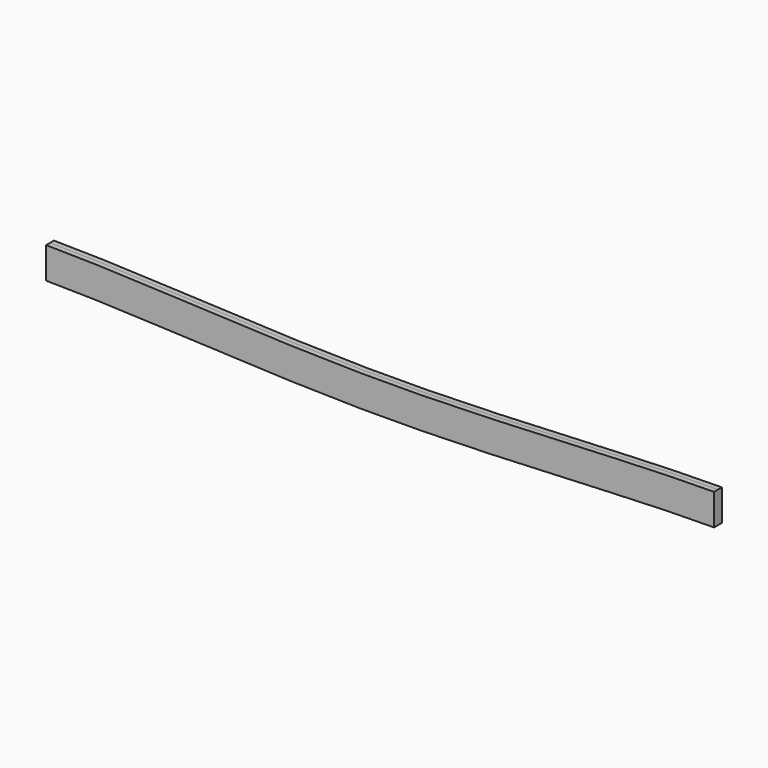
from build123d import *

# Parameters (mm, degrees)
F2_DEPTH = 23.8125


# Not quite as in the source:
# - a variable given as a bare number and used for a length is read in inches; the dataset says mm whatever the document's units were


with BuildPart() as f2:
    # F1 (on Front) → F2 (new body, symmetric)
    with BuildSketch(Plane.XZ):
        with BuildLine():
            Line((-1625.6, 76.2), (-1625.6, -76.2))
            add(Edge.make_bspline(
                [(-1625.6, -76.2), (-1188.0511561093, -76.2), (0, -177.8), (1188.0511561093, -76.2), (1625.6, -76.2)],
                knots=[0, 0, 0, 0, 0.5, 1, 1, 1, 1], degree=3))
            Line((1625.6, -76.2), (1625.6, 76.2))
            add(Edge.make_bspline(
                [(-1625.6, 76.2), (-1188.0511561093, 76.2), (0, -25.4), (1188.0511561093, 76.2), (1625.6, 76.2)],
                knots=[0, 0, 0, 0, 0.5, 1, 1, 1, 1], degree=3))
        make_face()
    extrude(amount=F2_DEPTH, both=True)


solid = f2.part
